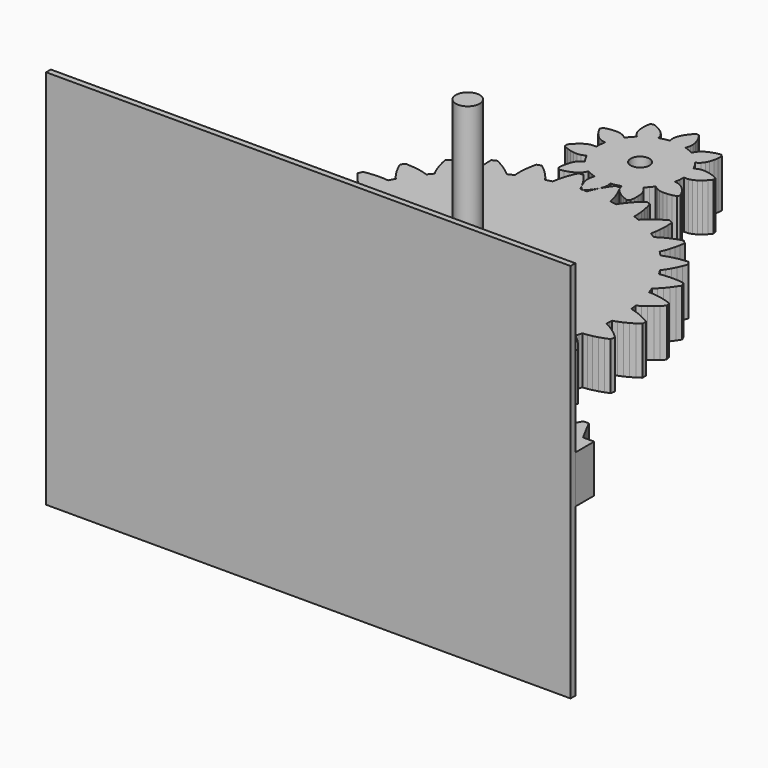
from build123d import *

# Parameters (mm, degrees)
F0_R     = 2.5
F1_DEPTH = 12.7
F0_R_2   = 3.175
F2_DEPTH = 50.8
F3_W     = 139.9607953856
F3_H     = 101.6
F4_DEPTH = 1.5875


# Not quite as in the source:
# - a length typed as a fraction of an inch, garbled in the dataset ("3 / 203.2 mm" for 3/8 in), is restored


with BuildPart() as f1:
    # F0 (on Top) → F1 (new body)
    with BuildSketch(Plane.XY):
        Polygon((-2.5705029119, 29.5798362145), (-1.7395310888, 30.4528103225), (-1.053036932, 31.3625053273), (-0.5197873049, 32.2948749843), (-0.1556223582, 33.2350704062), (-0.0138455841, 34.1644301536), (-0.1398002669, 35.3498328758), (1.1334215838, 35.560125225), (1.1339433015, 35.5580182883), (1.1531966897, 35.5634361256), (1.1731022251, 35.5667470261), (1.1726306726, 35.5689542931), (2.4142484727, 35.9207123925), (2.8050150002, 34.7945045587), (3.3290101586, 34.0139346747), (4.0588430001, 33.3182442409), (4.9382884137, 32.701714429), (5.946788717, 32.1708667097), (7.0703578634, 31.7348311421), (7.7731516839, 32.1504996549), (7.9323458014, 33.3451327665), (7.9530439463, 34.4845842024), (7.8364099502, 35.5522994601), (7.5783804351, 36.5270085119), (7.1468095667, 37.3622584198), (6.3481802253, 38.2471718358), (7.2545743626, 39.1657962391), (7.256269945, 39.1642912843), (7.2686908386, 39.1801434747), (7.2828073145, 39.1943903801), (7.2811317981, 39.1958953348), (8.0788782327, 40.210335193), (9.0569182511, 39.5288916645), (9.9396244, 39.2054267152), (10.9390147103, 39.0715860693), (12.0129504478, 39.0896455267), (13.1408638971, 39.2529832865), (14.3061002251, 39.5606963757), (14.630367817, 40.3100635304), (14.0569800424, 41.3700533535), (13.4039299942, 42.3041286259), (12.6819530167, 43.0993467365), (11.9003798296, 43.7362436032), (11.0603140663, 44.1582329261), (9.8939741048, 44.4047445205), (10.08731063, 45.680745521), (10.0896182274, 45.6805448604), (10.0904208699, 45.7007112546), (10.0933304492, 45.7204763275), (10.0911231821, 45.7206769881), (10.1402850386, 47.0102225817), (11.3321089012, 47.0339005371), (12.2363860688, 47.2910471454), (13.1235067518, 47.7701244199), (13.9817323029, 48.4160510154), (14.7981201108, 49.2111687956), (15.5600285554, 50.1449430771), (15.3819422387, 50.9417664728), (14.2949635597, 51.4623804995), (13.2176165913, 51.8342046627), (12.1661548453, 52.0531254193), (11.1594404218, 52.1090094072), (10.2316859594, 51.9566076522), (9.143302656, 51.4705072553), (8.5497585202, 52.6164801621), (8.5516948953, 52.6175837956), (8.5404679326, 52.6343389589), (8.5312475763, 52.6521977557), (8.5293112011, 52.6510941222), (7.8110765445, 53.723223914), (8.7614454608, 54.4427929638), (9.3418563578, 55.1823277471), (9.7778919254, 56.0914207701), (10.0925278066, 57.1184019182), (10.2857640015, 58.2415998424), (10.3531859761, 59.4448613615), (9.7407697072, 59.9848391398), (8.5554071172, 59.767122347), (7.4653181983, 59.4346276689), (6.4858835885, 58.993776246), (5.6386241413, 58.4471766666), (4.977668064, 57.7786757493), (4.382799568, 56.7455744517), (3.2290811606, 57.3237780817), (3.2299540344, 57.3258850184), (3.2110919344, 57.3328078104), (3.1931328072, 57.3418375392), (3.1922198013, 57.3397306025), (1.9809519228, 57.7849965594), (2.3267905334, 58.9257522895), (2.3616653523, 59.8652453992), (2.1801276726, 60.8570106052), (1.8310483928, 61.8728550879), (1.3271594303, 62.8950203806), (0.6744705713, 63.9081559446), (-0.1384157085, 63.9850089692), (-0.9693875316, 63.1121351915), (-1.6558816884, 62.2024401867), (-2.1891313155, 61.2700705297), (-2.5532962621, 60.3298751078), (-2.6950730363, 59.4005153603), (-2.5691183535, 58.2151126381), (-3.8423402042, 58.0047199586), (-3.8428619218, 58.0069272256), (-3.8621153101, 58.0014090581), (-3.8820208454, 57.9981984879), (-3.8815492929, 57.9959912208), (-5.123167093, 57.6442331215), (-5.5139336205, 58.770340625), (-6.037928779, 59.5509105089), (-6.7677616205, 60.2466009428), (-7.6472070341, 60.863231085), (-8.6557073373, 61.393978474), (-9.7792764838, 61.8300140415), (-10.4820703042, 61.4143455288), (-10.6412644218, 60.2197124172), (-10.6619625667, 59.0802609812), (-10.5453285705, 58.0125457235), (-10.2872990554, 57.0378366718), (-9.8557281871, 56.2026870941), (-9.0570988457, 55.3176733478), (-9.963492983, 54.3991492749), (-9.9651885654, 54.4005538994), (-9.9776094589, 54.3848020392), (-9.9917259348, 54.3704548036), (-9.9900504185, 54.3689498488), (-10.7877968531, 53.354610321), (-11.7658368714, 54.0360538495), (-12.6485430204, 54.3595187988), (-13.6479333307, 54.4933594447), (-14.7218690682, 54.4751996569), (-15.8497825174, 54.3118618971), (-17.0150188455, 54.0042491382), (-17.3392864374, 53.2548819836), (-16.7658986627, 52.1947918302), (-16.1128486146, 51.260816888), (-15.3908716371, 50.4655987775), (-14.60929845, 49.8287019107), (-13.7692326867, 49.4066122576), (-12.6028927251, 49.1601006631), (-12.7962292504, 47.8841999929), (-12.7985368477, 47.8844006536), (-12.7993394903, 47.8642342594), (-12.8022490695, 47.8444691865), (-12.8000418025, 47.8441681955), (-12.849203659, 46.5546226019), (-14.0410275216, 46.5310449769), (-14.9453046892, 46.2738983686), (-15.8324253722, 45.7947207637), (-16.6906509233, 45.1488944986), (-17.5070387312, 44.3537767183), (-18.2689471758, 43.4199021066), (-18.090860859, 42.6230787109), (-17.00388218, 42.1025650145), (-15.9265352117, 41.7307408513), (-14.8750734657, 41.5117197643), (-13.8683590421, 41.4559361068), (-12.9406045798, 41.6082375314), (-11.8522212763, 42.0943379283), (-11.2586771406, 40.9484653519), (-11.2606135157, 40.9472613881), (-11.249386553, 40.9305062248), (-11.2401661966, 40.9127477582), (-11.2382298215, 40.9138513918), (-10.5199951649, 39.8417216), (-11.4703640812, 39.1220522199), (-12.0507749782, 38.3825174365), (-12.4868105457, 37.4734244136), (-12.801446427, 36.4464432655), (-12.9946826219, 35.3233456716), (-13.0621045965, 34.1199838222), (-12.4496883276, 33.5800060439), (-11.2643157045, 33.797823167), (-10.1742267856, 34.1302175148), (-9.1948022089, 34.5710689376), (-8.3475427617, 35.117668517), (-7.6865666183, 35.7862697647), (-7.0917181884, 36.8192707319), (-5.9380198471, 36.2410671019), (-5.9388726548, 36.2389601652), (-5.9200607199, 36.2321377035), (-5.9020413946, 36.2230076445), (-5.9011183556, 36.2251145812), (-4.6898705432, 35.7799489546), (-5.0357091537, 34.6390928941), (-5.0705839727, 33.6997001148), (-4.889046293, 32.7078345784), (-4.5399670132, 31.6920904261), (-4.0360780507, 30.6699251334), (-3.3833891917, 29.656689239), align=None)
        with Locations((-1.3544593102, 46.7824225918)):
            Circle(F0_R, mode=Mode.SUBTRACT)
    extrude(amount=F1_DEPTH)


with BuildPart() as f1b:
    # F0 (on Top) → F1, piece 2 (new body)
    with BuildSketch(Plane.XY):
        Polygon((-4.1149778138, -56.6076202627), (-3.3087835663, -55.4982679225), (-2.5861343756, -54.3738660344), (-1.9511046561, -53.2373241777), (-1.4095416588, -52.0917525923), (-0.9706577134, -50.940261518), (-0.0671209836, -50.9209980967), (0.7890277299, -50.8849795121), (1.2993779649, -52.0066724815), (1.9118042668, -53.1159244914), (2.6169257506, -54.210327614), (3.4087627294, -55.2871729308), (4.2830310985, -56.343751523), (5.4895031878, -56.1785074872), (6.0474400933, -54.9256827904), (6.5205075817, -53.6755670123), (6.9053746864, -52.4318723746), (7.1969145281, -51.1988127507), (7.3868297895, -49.981203996), (8.2666062931, -49.7745235383), (9.0965487272, -49.5612212796), (9.8289600579, -50.5522841733), (10.658591468, -51.5099370708), (11.5759115771, -52.433878981), (12.5742985841, -53.3226049491), (13.6491372945, -54.1743090294), (14.7949095406, -53.7617507566), (15.0802489686, -52.4204347182), (15.2830165439, -51.0991847437), (15.400904669, -49.8027163581), (15.4296994707, -48.5358454166), (15.3622774961, -47.305394381), (16.1798692679, -46.9203266157), (16.9473962103, -46.5391717327), (17.8698331657, -47.3562618529), (18.8804604717, -48.1205782251), (19.9697467481, -48.8335254739), (21.131170524, -49.4953042598), (22.3596149531, -50.1049112797), (23.3945221964, -49.4631985576), (23.3947228571, -48.0917834235), (23.3183714841, -46.7572898468), (23.1641637834, -45.4646340133), (22.9288891847, -44.2195347512), (22.6071298508, -43.0299181555), (23.3267992309, -42.4833185761), (23.9983100578, -41.9508655718), (25.0704398496, -42.558365655), (26.2179177111, -43.0958351753), (27.4316135833, -43.566785694), (28.7052066562, -43.9725215051), (30.0335800834, -44.31344393), (30.9124736802, -43.4705689178), (30.6275355735, -42.1291525491), (30.2754764831, -40.8397072858), (29.8557947576, -39.6072496439), (29.3667847815, -38.438301094), (28.8048346632, -37.341590374), (29.3950779315, -36.6572372663), (29.9411758593, -35.9969634352), (31.1161442283, -36.3681856165), (32.3503074857, -36.6553309902), (33.6354385453, -36.863616733), (34.9656179182, -36.9957517635), (36.3357287582, -37.0530403758), (37.0202825266, -36.0458243006), (36.4625462817, -34.7928992736), (35.8501300129, -33.604887963), (35.183334711, -32.4867065548), (34.4620600458, -31.4448765194), (33.6842994108, -30.4890295677), (34.1193316751, -29.6969216971), (34.5162384182, -28.9374211802), (35.7427765713, -29.0563126085), (37.0096475127, -29.0805925458), (38.3100287808, -29.0170834537), (39.6385025383, -28.869798545), (40.9906542512, -28.6409450867), (41.4507690953, -27.5134329587), (40.6449159709, -26.4038799579), (39.7987300582, -25.3691733752), (38.9141176332, -24.4140287357), (37.9919816687, -23.5449675102), (37.0324224952, -22.7717217396), (37.2933816556, -21.9064730662), (37.5236397384, -21.0810555295), (38.7480709548, -20.9422986979), (39.9923675744, -20.7026095652), (41.25111176, -20.3701851184), (42.5198889775, -19.9498713118), (43.7948866748, -19.4448987819), (44.0105968613, -18.24639292), (42.9915418084, -17.3286313575), (41.9488088002, -16.4923881794), (40.8849060946, -15.7420478206), (39.8022416194, -15.0837103646), (38.7029223111, -14.5268369605), (38.7781700506, -13.6262619817), (38.8318467714, -12.7710262742), (40.0006949909, -12.3807212661), (41.1679379253, -11.8876077799), (42.3300640135, -11.3007315972), (43.4837623548, -10.6258105427), (44.6259227094, -9.8667655255), (44.5876968577, -8.64962732), (43.4000868685, -7.9637893235), (42.2062563995, -7.3626301165), (41.0096166815, -6.8498920198), (39.8136792758, -6.4310330029), (38.6226580557, -6.1148921669), (38.5090841343, -5.2183404339), (38.3837715655, -4.3706595994), (39.4458683253, -3.7458625691), (40.4850897723, -3.02083555), (41.4998306215, -2.2051701203), (42.487983936, -1.3051168592), (43.4473424489, -0.3252207299), (43.1568861746, 0.8573727433), (41.8526923544, 1.2813686726), (40.5599361905, 1.621187464), (39.2828315565, 1.8739195382), (38.025993647, 2.0349497007), (36.7952416204, 2.0965525167), (36.4977622238, 2.9498618821), (36.1988782027, 3.7530060879), (37.1079712256, 4.5850454256), (37.9737215506, 5.5102916299), (38.7966308293, 6.5190126599), (39.5760970797, 7.6048877054), (40.3108160078, 8.7629002505), (39.780770931, 9.8592096491), (38.4168805709, 10.002782336), (37.0817850123, 10.0663917584), (35.7799991197, 10.04803131), (34.517141391, 9.9442897599), (33.3004356092, 9.7486456373), (32.8319933485, 10.5214900867), (32.3727814772, 11.2448716886), (33.0889392962, 12.2476732298), (33.7433939688, 13.3327456327), (34.338653753, 14.4905575171), (34.8753206308, 15.7147880729), (35.3531939415, 17.0002201234), (34.6068366965, 17.9623878852), (33.2429463363, 17.8192165196), (31.9237029682, 17.6038073241), (30.6542234384, 17.3152573259), (29.4405275661, 16.9512589276), (28.2911434286, 16.5068959435), (27.672205689, 17.1654641592), (27.072631701, 17.7775794371), (27.5646515867, 18.9073991624), (27.9792164659, 20.1047411927), (28.3207408727, 21.3610774506), (28.5911310832, 22.6700871261), (28.7912900701, 24.0267537033), (27.8612280105, 24.8127414245), (26.5568335296, 24.3891468166), (25.3113329462, 23.9042503835), (24.1295421154, 23.3580521254), (23.0180828385, 22.749548739), (21.9860851745, 22.0759309754), (21.2438414725, 22.5914281558), (20.5299912509, 23.0655892447), (20.776402515, 24.2729643068), (20.9330181434, 25.5304041983), (21.0058579552, 26.8301834845), (20.9981325206, 28.1668843281), (20.911848446, 29.5354902133), (19.8387153511, 30.1109849247), (18.6510050315, 29.4254278531), (17.5334256052, 28.6921135495), (16.4909935879, 27.9121456475), (15.5303307809, 27.0859254683), (14.6610688947, 26.2124497087), (13.8278255931, 26.5624018623), (13.0310021975, 26.8776397255), (13.0209691656, 28.1098967068), (12.9127127511, 29.3724534445), (12.7136573976, 30.6589891286), (12.4283179696, 31.9647882339), (12.0593030553, 33.2856368871), (10.8899531842, 33.6254556785), (9.8706974707, 32.7079349087), (8.9301007275, 31.7582081065), (8.0726176208, 30.7785828691), (7.3047094232, 29.7706644817), (6.6359877792, 28.7355565778), (5.748194883, 28.9046131658), (4.9032630992, 29.0473832101), (4.6372874229, 30.2506447291), (4.2688644575, 31.4630363072), (3.8066828087, 32.68004308), (3.2560399174, 33.898053156), (2.6205577082, 35.1133543133), (1.4060591934, 35.2024476368), (0.5998649459, 34.0930952966), (-0.1227842447, 32.9686934085), (-0.7578139642, 31.8321515518), (-1.2993769616, 30.6865799664), (-1.7382609069, 29.5350888921), (-2.6417976368, 29.5158254708), (-3.4979463502, 29.4798068861), (-4.0082965853, 30.6014998556), (-4.6207228871, 31.7107518655), (-5.325844371, 32.8051549881), (-6.1176813498, 33.8820003049), (-6.9919497189, 34.9385788971), (-8.1984318412, 34.7733348613), (-8.7563787797, 33.5205101645), (-9.2294462681, 32.2703943864), (-9.6143033398, 31.0266997487), (-9.9058532146, 29.7936401248), (-10.0957584429, 28.5760313701), (-10.9755349465, 28.3693509124), (-11.8054673476, 28.1560486537), (-12.5378786783, 29.1471115474), (-13.3675100883, 30.1047644449), (-14.2848301974, 31.0287063551), (-15.2832172045, 31.9174323232), (-16.3580559149, 32.7691364035), (-17.503828161, 32.3565781307), (-17.789167589, 31.0152620923), (-17.9919351642, 29.6940121178), (-18.1098232894, 28.3975437321), (-18.138618091, 27.1306727907), (-18.0711961165, 25.9002217551), (-18.8887878882, 25.5151539898), (-19.6563148307, 25.1339991068), (-20.5787517861, 25.951089227), (-21.5893790921, 26.7154055992), (-22.6786653684, 27.428352848), (-23.8400891443, 28.0901316339), (-25.0685335735, 28.6997386538), (-26.1034408168, 28.0580259317), (-26.1036414775, 26.6866107976), (-26.0272901045, 25.3521172209), (-25.8730824038, 24.0594613874), (-25.6378078051, 22.8143621253), (-25.3160484712, 21.6247455296), (-26.0357178513, 21.0781459502), (-26.7072286782, 20.5456929459), (-27.7793584699, 21.1531930291), (-28.9268363315, 21.6906625494), (-30.1405322037, 22.1616130681), (-31.4141252766, 22.5673488792), (-32.7424987037, 22.9082713041), (-33.6213923006, 22.0653962919), (-33.3364541938, 20.7239799232), (-32.9843951035, 19.4345346599), (-32.564713378, 18.202077018), (-32.0757034019, 17.0331284681), (-31.5137532836, 15.9364177481), (-32.1039965519, 15.2520646404), (-32.6500944797, 14.5917908092), (-33.8250628487, 14.9630129906), (-35.0592261061, 15.2501583643), (-36.3443571656, 15.4584441071), (-37.6745365386, 15.5905791376), (-39.0446473785, 15.6478677499), (-39.7292011469, 14.6406516747), (-39.1714649021, 13.3877266477), (-38.5590486333, 12.1997153371), (-37.8922533314, 11.0815339288), (-37.1709786661, 10.0397038935), (-36.3932180311, 9.0838569418), (-36.8282502955, 8.2917490711), (-37.2251570385, 7.5322485542), (-38.4516951916, 7.6511399826), (-39.7185661331, 7.6754199199), (-41.0189474012, 7.6119108278), (-42.3474211587, 7.4646259191), (-43.6995728715, 7.2357724608), (-44.1596877157, 6.1082603328), (-43.3538345913, 4.998707332), (-42.5076486786, 3.9640007493), (-41.6230362535, 3.0088561098), (-40.7009002891, 2.1397948843), (-39.7413411156, 1.3665491137), (-40.002300276, 0.5013004402), (-40.2325583587, -0.3241170964), (-41.4569895751, -0.462873928), (-42.7012861948, -0.7025630607), (-43.9600303804, -1.0349875076), (-45.2288075979, -1.4553013141), (-46.5038052952, -1.960273844), (-46.7195154816, -3.1587797059), (-45.7004604288, -4.0765412684), (-44.6577274206, -4.9127844465), (-43.593824715, -5.6631248053), (-42.5111602397, -6.3214622613), (-41.4118409315, -6.8783356654), (-41.4870886709, -7.7789106442), (-41.5407653917, -8.6341463517), (-42.7096136113, -9.0244513598), (-43.8768565457, -9.517564846), (-45.0389826338, -10.1044410287), (-46.1926809751, -10.7793620832), (-47.3348413297, -11.5384071004), (-47.2966154781, -12.7555453059), (-46.1090054889, -13.4413833024), (-44.9151750198, -14.0425425094), (-43.7185353019, -14.5552806061), (-42.5225978961, -14.974139623), (-41.331576676, -15.290280459), (-41.2180027546, -16.186832192), (-41.0926901859, -17.0345130265), (-42.1547869457, -17.6593100568), (-43.1940083927, -18.384337076), (-44.2087492418, -19.2000025056), (-45.1969025564, -20.1000557667), (-46.1562610692, -21.079951896), (-45.8658047949, -22.2625453693), (-44.5616109747, -22.6865412985), (-43.2688548109, -23.0263600899), (-41.9917501769, -23.2790921641), (-40.7349122673, -23.4401223266), (-39.5041602408, -23.5017251426), (-39.2066808442, -24.355034508), (-38.9077968231, -25.1581787138), (-39.816889846, -25.9902180515), (-40.682640171, -26.9154642558), (-41.5055494497, -27.9241852858), (-42.2850157001, -29.0100603313), (-43.0197346281, -30.1680728764), (-42.4896895514, -31.2643822751), (-41.1257991912, -31.4079549619), (-39.7907036327, -31.4715643843), (-38.4889177401, -31.4532039359), (-37.2260600114, -31.3494623858), (-36.0093542296, -31.1538182632), (-35.5409119689, -31.9266627126), (-35.0817000976, -32.6500443145), (-35.7978579166, -33.6528458557), (-36.4523125892, -34.7379182586), (-37.0475723734, -35.895730143), (-37.5842392512, -37.1199606988), (-38.0621125619, -38.4053927493), (-37.3157553168, -39.3675605111), (-35.9518649566, -39.2243891455), (-34.6326215885, -39.00897995), (-33.3631420588, -38.7204299518), (-32.1494461865, -38.3564315535), (-31.0000620489, -37.9120685694), (-30.3811243093, -38.5706367851), (-29.7815503214, -39.182752063), (-30.2735702071, -40.3125717884), (-30.6881350863, -41.5099138186), (-31.0296594931, -42.7662500765), (-31.3000497036, -44.075259752), (-31.5002086905, -45.4319263293), (-30.5701466308, -46.2179140504), (-29.26575215, -45.7943194425), (-28.0202515665, -45.3094230094), (-26.8384607358, -44.7632247513), (-25.7270014589, -44.1547213649), (-24.6950037949, -43.4811036013), (-23.9527600929, -43.9966007817), (-23.2389098713, -44.4707618706), (-23.4853211354, -45.6781369327), (-23.6419367638, -46.9355768242), (-23.7147765756, -48.2353561104), (-23.707051141, -49.572056954), (-23.6207670664, -50.9406628392), (-22.5476339715, -51.5161575506), (-21.3599236519, -50.830600479), (-20.2423442255, -50.0972861754), (-19.1999122083, -49.3173182734), (-18.2392494013, -48.4910980942), (-17.3699875151, -47.6176223346), (-16.5367442135, -47.9675744882), (-15.7399208178, -48.2828123514), (-15.7298877859, -49.5150693327), (-15.6216313714, -50.7776260704), (-15.422576018, -52.0641617545), (-15.13723659, -53.3699608598), (-14.7682216757, -54.690809513), (-13.5988718046, -55.0306283044), (-12.5796160911, -54.1131075347), (-11.6390193479, -53.1633807324), (-10.7815362412, -52.183755495), (-10.0136280435, -51.1758371076), (-9.3449063995, -50.1407292037), (-8.4571135034, -50.3097857917), (-7.6121817196, -50.452555836), (-7.3462060432, -51.655817355), (-6.9777830778, -52.8682089331), (-6.5156014291, -54.0852157059), (-5.9649585378, -55.3032257819), (-5.3294763286, -56.5185269392), align=None)
        with Locations((-1.3544593102, -10.702586313)):
            Circle(F0_R_2, mode=Mode.SUBTRACT)
    extrude(amount=F1_DEPTH)


with BuildPart() as f1c:
    # F0 (on Top) → F1, piece 3 (new body)
    with BuildSketch(Plane.XY):
        Polygon((69.9803976928, -63.9850089692), (69.9803976928, -57.6938966295), (66.9999852285, -57.6938966295), (63.9309810923, -51.9454709868), (62.4852211915, -51.9454709868), (59.416116725, -57.6938966295), (57.9702564939, -57.6938966295), (54.9012523577, -51.9454709868), (53.455492457, -51.9454709868), (50.3863879904, -57.6938966295), (48.9405277594, -57.6938966295), (45.8715236231, -51.9454709868), (44.4257637224, -51.9454709868), (41.3566592559, -57.6938966295), (39.9107990248, -57.6938966295), (36.8417948886, -51.9454709868), (35.3960349879, -51.9454709868), (32.3269305213, -57.6938966295), (30.8810702903, -57.6938966295), (27.812066154, -51.9454709868), (26.3663062533, -51.9454709868), (23.2972017868, -57.6938966295), (21.8513415557, -57.6938966295), (18.7823374195, -51.9454709868), (17.3365775188, -51.9454709868), (14.2674730522, -57.6938966295), (12.8216128212, -57.6938966295), (9.7526086849, -51.9454709868), (8.3068086521, -51.9454709868), (5.2377844498, -57.6938966295), (3.7919242187, -57.6938966295), (0.7229100495, -51.9454709868), (-0.7229240957, -51.9454709868), (-3.7919242187, -57.6938966295), (-5.2377844498, -57.6938966295), (-8.3068086521, -51.9454709868), (-9.752638784, -51.9454709868), (-12.8216128212, -57.6938966295), (-14.2674730522, -57.6938966295), (-17.3365775188, -51.9454709868), (-18.7823374195, -51.9454709868), (-21.8513415557, -57.6938966295), (-23.2972017868, -57.6938966295), (-26.3663062533, -51.9454709868), (-27.812066154, -51.9454709868), (-30.8810702903, -57.6938966295), (-32.3269305213, -57.6938966295), (-35.3960349879, -51.9454709868), (-36.8417948886, -51.9454709868), (-39.9107990248, -57.6938966295), (-41.3566592559, -57.6938966295), (-44.4257637224, -51.9454709868), (-45.8715236231, -51.9454709868), (-48.9405277594, -57.6938966295), (-50.3863879904, -57.6938966295), (-53.455492457, -51.9454709868), (-54.9012523577, -51.9454709868), (-57.9702564939, -57.6938966295), (-59.416116725, -57.6938966295), (-62.4852211915, -51.9454709868), (-63.9309810923, -51.9454709868), (-66.9999852285, -57.6938966295), (-69.9803976928, -57.6938966295), (-69.9803976928, -63.9850089692), align=None)
    extrude(amount=F1_DEPTH)


with BuildPart() as f2:
    # F0 (on Top) → F2 (new body)
    with BuildSketch(Plane.XY):
        with Locations((-1.3544593102, -10.702586313)):
            Circle(F0_R_2)
    extrude(amount=F2_DEPTH)


with BuildPart() as f4:
    # F3 (on face) → F4 (new body)
    with BuildSketch(Plane.XZ.offset(63.9850089692)):
        with Locations((0, 6.35)):
            Rectangle(F3_W, F3_H)
    extrude(amount=F4_DEPTH)


solid = Compound([f1.part, f1b.part, f1c.part, f2.part, f4.part])
